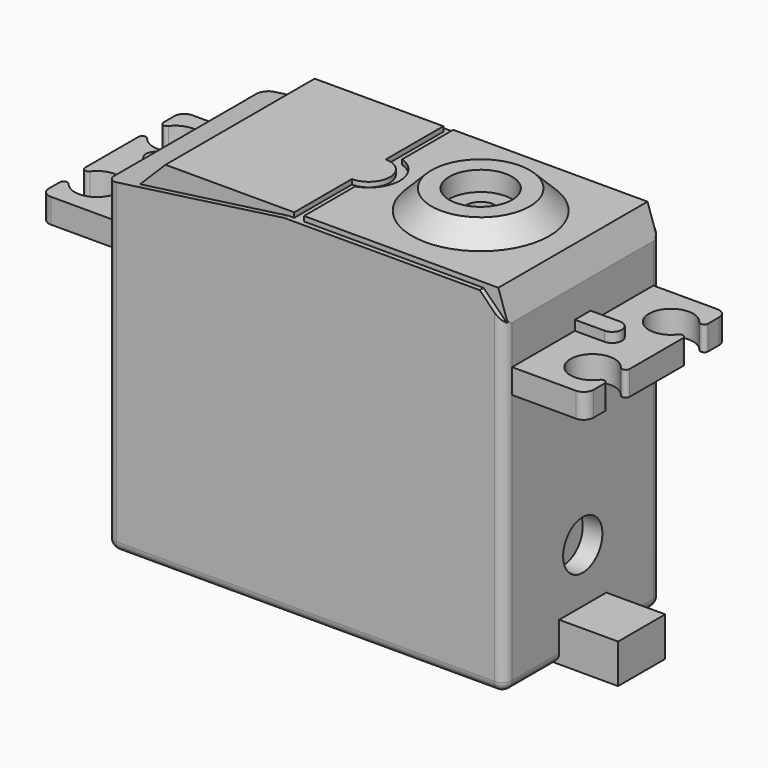
from build123d import *

# Parameters (mm, degrees)
F1_DEPTH      = 20
F2_W          = 7.5
F2_H          = 1
F3_DEPTH      = 2.5
F5_DEPTH      = 1
F7_DEPTH      = 20
F10_DEPTH     = 19
F12_DEPTH     = 0.5
F14_DEPTH     = 0.5
F15_R         = 7
F15_R_2       = 3.2
F16_DEPTH     = 2
F17_SIZE      = 1.99999
F18_R         = 1.5
F19_DEPTH     = 2
F20_R         = 2.5
F21_DEPTH     = 2
F22_W         = 6
F22_H         = 4
F23_DEPTH     = 6
F24_T1_DEPTH  = 34.6
F24_T3_DEPTH  = 7.5
F24_T5_DEPTH  = 38.5
F24_T7_DEPTH  = 18
F24_T9_DEPTH  = 6
F24_T11_DEPTH = 6
F24_S15_W     = 1
F24_S15_H     = 1
F24_T16_DEPTH = 1
F24_S21_W     = 1
F24_S21_H     = 1
F24_T22_DEPTH = 1
F24_S27_W     = 1
F24_S27_H     = 1
F24_T28_DEPTH = 1
F24_S33_W     = 1
F24_S33_H     = 1
F24_T34_DEPTH = 1


# Not quite as in the source:
# - a fillet or chamfer that OpenCascade refuses, or shapes differently, is made with other operations: its cross-section is extruded or revolved along the edge and cut away or added
# - a fillet or chamfer is up to 0.001 mm smaller than in the source, because OpenCascade refuses the exact size


with BuildPart() as f1:
    # F0 (on Front) → F1 (new body)
    with BuildSketch(Plane.XZ):
        Polygon((0, 26.6), (0, 0), (40.5, 0), (40.5, 26.6), (48, 26.6), (48, 29.1), (40.5, 29.1), (40.5, 36.1), (0, 36.1), (0, 29.1), (-7.5, 29.1), (-7.5, 26.6), align=None)
    extrude(amount=F1_DEPTH)

    # F2 (on face) → F3 (cut, through all)
    with BuildSketch(Plane.XY.offset(29.1)):
        with Locations((-3.75, -0.5)):
            Rectangle(F2_W, F2_H)
        with Locations((-3.75, -19.5)):
            Rectangle(F2_W, F2_H)
        with BuildLine():
            ThreePointArc((-7.5, -6.6), (-7.2314497593, -6.2261647771), (-6.7914469101, -6.3613294855))
            ThreePointArc((-6.7914469101, -6.3613294855), (-2.75, -5), (-6.7914469101, -3.6386705145))
            ThreePointArc((-6.7914469101, -3.6386705145), (-7.2314497593, -3.7738352229), (-7.5, -3.4))
            Line((-7.5, -3.4), (-7.5, -6.6))
        make_face()
        with BuildLine():
            ThreePointArc((-7.5, -16.6), (-7.2314497593, -16.2261647771), (-6.7914469101, -16.3613294855))
            ThreePointArc((-6.7914469101, -16.3613294855), (-2.75, -15), (-6.7914469101, -13.6386705145))
            ThreePointArc((-6.7914469101, -13.6386705145), (-7.2314497593, -13.7738352229), (-7.5, -13.4))
            Line((-7.5, -13.4), (-7.5, -16.6))
        make_face()
        with BuildLine():
            Line((48, -16.6), (48, -13.4))
            ThreePointArc((48, -13.4), (47.7314497593, -13.7738352229), (47.2914469101, -13.6386705145))
            ThreePointArc((47.2914469101, -13.6386705145), (43.25, -15), (47.2914469101, -16.3613294855))
            ThreePointArc((47.2914469101, -16.3613294855), (47.7314497593, -16.2261647771), (48, -16.6))
        make_face()
        with Locations((44.25, -0.5)):
            Rectangle(F2_W, F2_H)
        with BuildLine():
            ThreePointArc((47.2914469101, -3.6386705145), (43.25, -5), (47.2914469101, -6.3613294855))
            ThreePointArc((47.2914469101, -6.3613294855), (47.7314497593, -6.2261647771), (48, -6.6))
            Line((48, -6.6), (48, -3.4))
            ThreePointArc((48, -3.4), (47.7314497593, -3.7738352229), (47.2914469101, -3.6386705145))
        make_face()
        with Locations((44.25, -19.5)):
            Rectangle(F2_W, F2_H)
    extrude(amount=-F3_DEPTH, mode=Mode.SUBTRACT)

    # F4 (on face) → F5 (join)
    with BuildSketch(Plane.XY.offset(29.1)):
        with BuildLine():
            Line((0, -11), (0, -9))
            Line((0, -9), (-3, -9))
            ThreePointArc((-3, -9), (-4, -10), (-3, -11))
            Line((-3, -11), (0, -11))
        make_face()
        with BuildLine():
            Line((43.5, -9), (40.5, -9))
            Line((40.5, -9), (40.5, -11))
            Line((40.5, -11), (43.5, -11))
            ThreePointArc((43.5, -11), (44.5, -10), (43.5, -9))
        make_face()
    extrude(amount=F5_DEPTH)

    # F6 (on face) → F7 (cut, through all)
    with BuildSketch(Plane.XZ.offset(20)):
        Polygon((40.5, 36.1), (0, 36.1), (0, 33.1), (18.1, 35.6), (38, 35.6), (40.5, 33.1), align=None)
    extrude(amount=-F7_DEPTH, mode=Mode.SUBTRACT)

    # F9 (on offset) → F10 (join)
    with BuildSketch(Plane.XZ.offset(19.5)):
        Polygon((5.5856353591, 36.1), (3, 33.5143646409), (18.1, 35.6), (18.7, 35.6), (18.7, 36.1), align=None)
        Polygon((39.5, 36.1), (19.7, 36.1), (19.7, 35.6), (38, 35.6), (40.5, 33.1), align=None)
    extrude(amount=-F10_DEPTH)

    # F11 (on face) → F12 (cut, through all)
    with BuildSketch(Plane.XY.offset(36.1)):
        with BuildLine():
            Line((19.7, -7), (19.7, -13))
            ThreePointArc((19.7, -13), (21.8622776602, -10), (19.7, -7))
        make_face()
    extrude(amount=-F12_DEPTH, mode=Mode.SUBTRACT)

    # F13 (on face) → F14 (join)
    with BuildSketch(Plane.XY.offset(35.6)):
        with BuildLine():
            Line((18.7, -7.8377223398), (18.7, -12.1622776602))
            ThreePointArc((18.7, -12.1622776602), (20.8622776602, -10), (18.7, -7.8377223398))
        make_face()
    extrude(amount=F14_DEPTH)

    # F15 (on face) → F16 (join)
    with BuildSketch(Plane.XY.offset(36.1)):
        with Locations((30.1, -10)):
            Circle(F15_R)
        with Locations((30.1, -10)):
            Circle(F15_R_2, mode=Mode.SUBTRACT)
    extrude(amount=F16_DEPTH)

    # F17 (size 2 in the source; OpenCascade refuses exactly that, so slightly less here)
    f17_edges = [f1.edges().sort_by_distance(p)[0] for p in [
        (23.1, -10, 38.1),
    ]]
    chamfer(f17_edges, length=F17_SIZE)

    # F18 (on face) → F19 (cut)
    with BuildSketch(Plane.XY.offset(36.1)):
        with Locations((30.1, -10)):
            Circle(F18_R)
    extrude(amount=-F19_DEPTH, mode=Mode.SUBTRACT)

    # F20 (on face) → F21 (cut)
    with BuildSketch(Plane.YZ.offset(40.5)):
        with Locations((-10, 9.5)):
            Circle(F20_R)
    extrude(amount=-F21_DEPTH, mode=Mode.SUBTRACT)

    # F22 (on face) → F23 (join)
    with BuildSketch(Plane.YZ.offset(40.5)):
        with Locations((-10, 2)):
            Rectangle(F22_W, F22_H)
    extrude(amount=F23_DEPTH)

    # F24: fillet of radius 1 on 13 edges, made by hand

    # F24_s2 → F24_t1 (cut)
    with BuildSketch(Plane.XY.offset(1)):
        with BuildLine():
            ThreePointArc((1, 0), (0.2928932188, -0.2928932188), (0, -1))
            Line((0, -1), (0, 0))
            Line((0, 0), (1, 0))
        make_face()
        with BuildLine():
            ThreePointArc((1, -20), (0.2928932188, -19.7071067812), (0, -19))
            Line((0, -19), (0, -20))
            Line((0, -20), (1, -20))
        make_face()
        with BuildLine():
            ThreePointArc((40.5, -19), (40.2071067812, -19.7071067812), (39.5, -20))
            Line((39.5, -20), (40.5, -20))
            Line((40.5, -20), (40.5, -19))
        make_face()
        with BuildLine():
            ThreePointArc((40.5, -1), (40.2071067812, -0.2928932188), (39.5, 0))
            Line((39.5, 0), (40.5, 0))
            Line((40.5, 0), (40.5, -1))
        make_face()
    extrude(amount=F24_T1_DEPTH, mode=Mode.SUBTRACT)

    # F24_s4 → F24_t3 (cut)
    with BuildSketch(Plane.XY.offset(24.1)):
        with BuildLine():
            ThreePointArc((-6.5, -19), (-7.2071067812, -18.7071067812), (-7.5, -18))
            Line((-7.5, -18), (-7.5, -19))
            Line((-7.5, -19), (-6.5, -19))
        make_face()
        with BuildLine():
            ThreePointArc((-6.5, -1), (-7.2071067812, -1.2928932188), (-7.5, -2))
            Line((-7.5, -2), (-7.5, -1))
            Line((-7.5, -1), (-6.5, -1))
        make_face()
        with BuildLine():
            ThreePointArc((47, -1), (47.7071067812, -1.2928932188), (48, -2))
            Line((48, -2), (48, -1))
            Line((48, -1), (47, -1))
        make_face()
        with BuildLine():
            ThreePointArc((47, -19), (47.7071067812, -18.7071067812), (48, -18))
            Line((48, -18), (48, -19))
            Line((48, -19), (47, -19))
        make_face()
    extrude(amount=F24_T3_DEPTH, mode=Mode.SUBTRACT)

    # F24_s6 → F24_t5 (cut)
    with BuildSketch(Plane.YZ.offset(1)):
        with BuildLine():
            ThreePointArc((-20, 1), (-19.7071067812, 0.2928932188), (-19, 0))
            Line((-19, 0), (-20, 0))
            Line((-20, 0), (-20, 1))
        make_face()
        with BuildLine():
            ThreePointArc((0, 1), (-0.2928932188, 0.2928932188), (-1, 0))
            Line((-1, 0), (0, 0))
            Line((0, 0), (0, 1))
        make_face()
    extrude(amount=F24_T5_DEPTH, mode=Mode.SUBTRACT)

    # F24_s8 → F24_t7 (cut)
    with BuildSketch(Plane.XZ.offset(1)):
        with BuildLine():
            ThreePointArc((1, 0), (0.2928932188, 0.2928932188), (0, 1))
            Line((0, 1), (0, 0))
            Line((0, 0), (1, 0))
        make_face()
    extrude(amount=F24_T7_DEPTH, mode=Mode.SUBTRACT)

    # F24_s10 → F24_t9 (cut)
    with BuildSketch(Plane.XZ.offset(13)):
        with BuildLine():
            ThreePointArc((40.5, 1), (40.2071067812, 0.2928932188), (39.5, 0))
            Line((39.5, 0), (40.5, 0))
            Line((40.5, 0), (40.5, 1))
        make_face()
    extrude(amount=F24_T9_DEPTH, mode=Mode.SUBTRACT)

    # F24_s12 → F24_t11 (cut)
    with BuildSketch(Plane.XZ.offset(1)):
        with BuildLine():
            ThreePointArc((40.5, 1), (40.2071067812, 0.2928932188), (39.5, 0))
            Line((39.5, 0), (40.5, 0))
            Line((40.5, 0), (40.5, 1))
        make_face()
    extrude(amount=F24_T11_DEPTH, mode=Mode.SUBTRACT)


with BuildPart() as f24_tool14:
    # F24_s15 → F24_t16 (new body)
    with BuildSketch(Plane.XY.offset(1)):
        with Locations((0.5, -0.5)):
            Rectangle(F24_S15_W, F24_S15_H)
    extrude(amount=-F24_T16_DEPTH)

    # F24_s17 → F24_t18 (revolve, cut)
    with BuildSketch(Plane(origin=(1, -1, 1), x_dir=(0.7071067812, -0.7071067812, 0), z_dir=(0.7071067812, 0.7071067812, 0))):
        with BuildLine():
            ThreePointArc((0, -1), (1, 0), (0, 1))
            Line((0, 1), (0, -1))
        make_face()
    revolve(axis=Axis((1, -1, 1), (0, 0, -1)), mode=Mode.SUBTRACT)


with BuildPart() as f1_1:
    add(f1.part)

    # F24_t13: cut F24_tool14
    add(f24_tool14.part, mode=Mode.SUBTRACT)


with BuildPart() as f24_tool20:
    # F24_s21 → F24_t22 (new body)
    with BuildSketch(Plane.XZ.offset(19)):
        with Locations((0.5, 0.5)):
            Rectangle(F24_S21_W, F24_S21_H)
    extrude(amount=F24_T22_DEPTH)

    # F24_s23 → F24_t24 (revolve, cut)
    with BuildSketch(Plane(origin=(1, -19, 1), x_dir=(0.7071067812, 0, 0.7071067812), z_dir=(0.7071067812, 0, -0.7071067812))):
        with BuildLine():
            ThreePointArc((0, -1), (1, 0), (0, 1))
            Line((0, 1), (0, -1))
        make_face()
    revolve(axis=Axis((1, -19, 1), (0, -1, 0)), mode=Mode.SUBTRACT)


with BuildPart() as f1_2:
    add(f1_1.part)

    # F24_t19: cut F24_tool20
    add(f24_tool20.part, mode=Mode.SUBTRACT)


with BuildPart() as f24_tool26:
    # F24_s27 → F24_t28 (new body)
    with BuildSketch(Plane.XZ.offset(19)):
        with Locations((40, 0.5)):
            Rectangle(F24_S27_W, F24_S27_H)
    extrude(amount=F24_T28_DEPTH)

    # F24_s29 → F24_t30 (revolve, cut)
    with BuildSketch(Plane(origin=(39.5, -19, 1), x_dir=(-0.7071067812, 0, 0.7071067812), z_dir=(0.7071067812, 0, 0.7071067812))):
        with BuildLine():
            ThreePointArc((0, -1), (1, 0), (0, 1))
            Line((0, 1), (0, -1))
        make_face()
    revolve(axis=Axis((39.5, -19, 1), (0, -1, 0)), mode=Mode.SUBTRACT)


with BuildPart() as f1_3:
    add(f1_2.part)

    # F24_t25: cut F24_tool26
    add(f24_tool26.part, mode=Mode.SUBTRACT)


with BuildPart() as f24_tool32:
    # F24_s33 → F24_t34 (new body)
    with BuildSketch(Plane.XY.offset(1)):
        with Locations((40, -0.5)):
            Rectangle(F24_S33_W, F24_S33_H)
    extrude(amount=-F24_T34_DEPTH)

    # F24_s35 → F24_t36 (revolve, cut)
    with BuildSketch(Plane(origin=(39.5, -1, 1), x_dir=(-0.7071067812, -0.7071067812, 0), z_dir=(0.7071067812, -0.7071067812, 0))):
        with BuildLine():
            ThreePointArc((0, -1), (1, 0), (0, 1))
            Line((0, 1), (0, -1))
        make_face()
    revolve(axis=Axis((39.5, -1, 1), (0, 0, -1)), mode=Mode.SUBTRACT)


with BuildPart() as f1_4:
    add(f1_3.part)

    # F24_t31: cut F24_tool32
    add(f24_tool32.part, mode=Mode.SUBTRACT)


solid = f1_4.part
